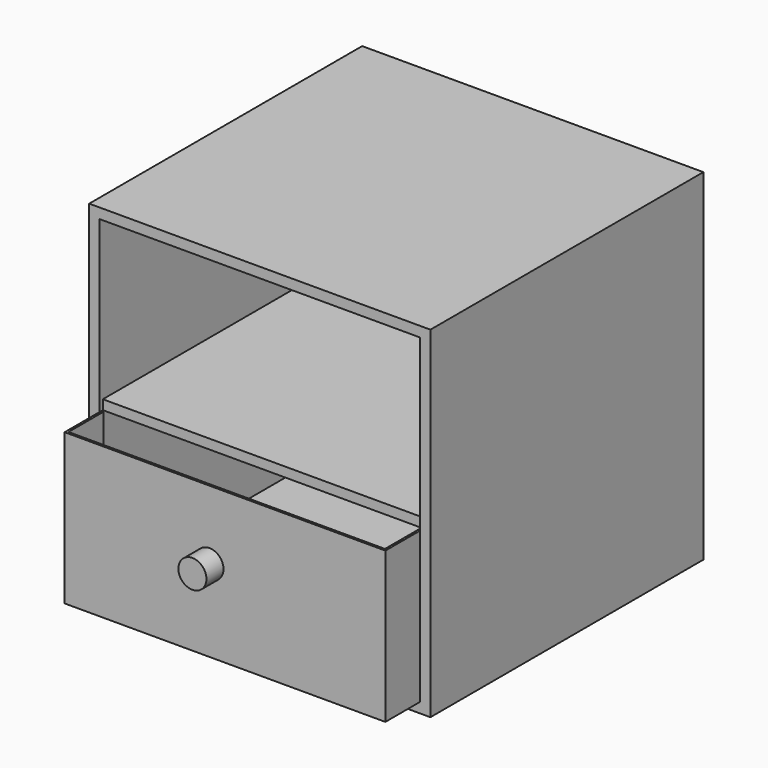
from build123d import *

# Parameters (mm, degrees)
F0_W      = 400
F0_H      = 400
F1_DEPTH  = 400
F2_T      = -12
F4_W      = 376
F4_H      = 11.2500011921
F5_DEPTH  = 383
F6_W      = 376
F6_H      = 176.7499988079
F7_DEPTH  = 439
F8_T      = -2.5
F9_R      = 16.4515915788
F10_DEPTH = 25


# Not quite as in the source:
# - a shell that OpenCascade refuses in one call is made with other operations: the cavity is built on its own and cut out


with BuildPart() as f1:
    # F0 (on Top) → F1 (new body)
    with BuildSketch(Plane.XY):
        with Locations((-4.0007606149, 88.9041203893)):
            Rectangle(F0_W, F0_H)
    extrude(amount=F1_DEPTH)

    # F2
    f2_openings = [f1.faces().sort_by_distance(p)[0] for p in [
        (-4.000761, -111.09588, 200),
    ]]
    offset(amount=F2_T, openings=f2_openings)

    # F4 (on face) → F5 (join)
    with BuildSketch(Plane.XZ.offset(-276.9041203893)):
        with Locations((-4.0007606149, 194.374999404)):
            Rectangle(F4_W, F4_H)
    extrude(amount=F5_DEPTH)

    # F6 (on face) → F7 (join)
    with BuildSketch(Plane.XZ.offset(-276.9041203893)):
        with Locations((-4.0007606149, 100.374999404)):
            Rectangle(F6_W, F6_H)
    extrude(amount=F7_DEPTH)

    # F8: a shell. OpenCascade refuses it in one call, so the cavity is built on its own and cut out:
    # the body offset inwards by the wall thickness, plus a prism from it out through each open face.
    f8_core = offset(f1.part, amount=F8_T, kind=Kind.INTERSECTION, mode=Mode.PRIVATE)
    f8_exits = [f8_core.faces().sort_by_distance(p)[0] for p in [
        (-4.000761, -131.534658, 186.249999),
    ]]
    add(f8_core, mode=Mode.SUBTRACT)
    extrude(f8_exits, amount=-F8_T, mode=Mode.SUBTRACT)

    # F9 (on face) → F10 (join)
    with BuildSketch(Plane.XZ.offset(162.0958796107)):
        with Locations((-22.2093164921, 107.9253256321)):
            Circle(F9_R)
    extrude(amount=F10_DEPTH)


solid = f1.part
